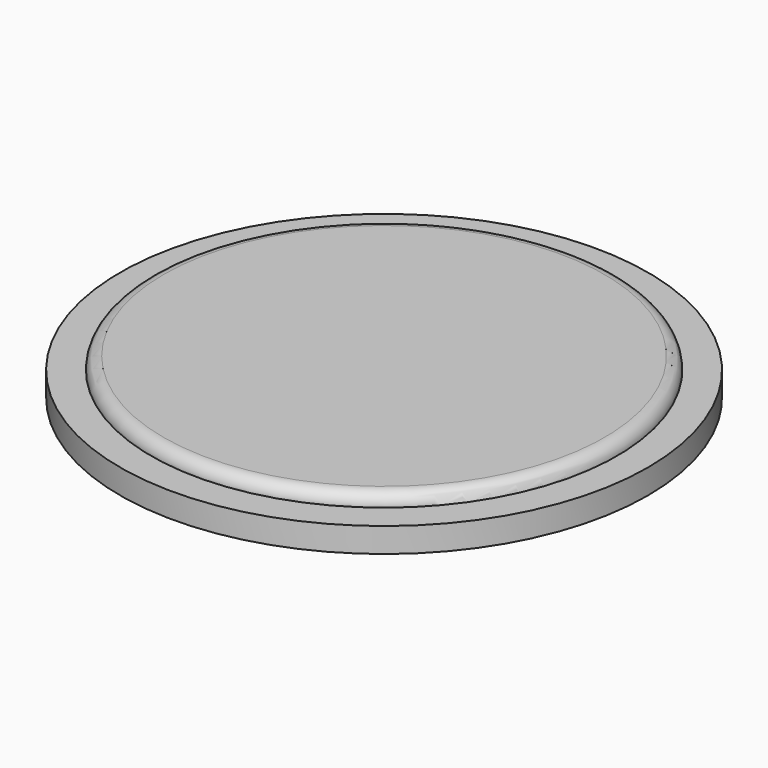
from build123d import *

# Parameters (mm, degrees)
F3_DEPTH = 2.38125
F4_DEPTH = 1.5875


# Not quite as in the source:
# - a fillet or chamfer that OpenCascade refuses, or shapes differently, is made with other operations: its cross-section is extruded or revolved along the edge and cut away or added


with BuildPart() as f3:
    # F2 (on Top) → F3 (new body)
    with BuildSketch(Plane.XY):
        with BuildLine():
            Line((-15, 0), (15, 0))
            ThreePointArc((15, 0), (0, 15), (-15, 0))
        make_face()
        with BuildLine():
            ThreePointArc((-15, 0), (0, -15), (15, 0))
            Line((15, 0), (-15, 0))
        make_face()
    extrude(amount=F3_DEPTH)

    # F2 (on Top) → F4 (join)
    with BuildSketch(Plane.XY):
        with BuildLine():
            Line((17, 0), (15, 0))
            ThreePointArc((15, 0), (0, -15), (-15, 0))
            Line((-15, 0), (-17, 0))
            ThreePointArc((-17, 0), (0, -17), (17, 0))
        make_face()
        with BuildLine():
            ThreePointArc((-15, 0), (0, 15), (15, 0))
            Line((15, 0), (17, 0))
            ThreePointArc((17, 0), (0, 17), (-17, 0))
            Line((-17, 0), (-15, 0))
        make_face()
    extrude(amount=F4_DEPTH)

    # F5: fillet of radius 0.7971733183 on 1 edges, made by hand


with BuildPart() as f5_tool2:
    # F5_s3 → F5_t4 (revolve)
    with BuildSketch(Plane.XZ):
        with BuildLine():
            ThreePointArc((-15, 1.5840766817), (-14.7665133409, 2.1477633409), (-14.2028266817, 2.38125))
            Line((-14.2028266817, 2.38125), (-15, 2.38125))
            Line((-15, 2.38125), (-15, 1.5840766817))
        make_face()
    revolve(axis=Axis((0, 0, 2.38125), (0, 0, 1)))

    split(bisect_by=Plane.XY.offset(1.5875), keep=Keep.TOP)


with BuildPart() as f3_1:
    add(f3.part)

    # F5_t1: cut F5_tool2
    add(f5_tool2.part, mode=Mode.SUBTRACT)


solid = f3_1.part
